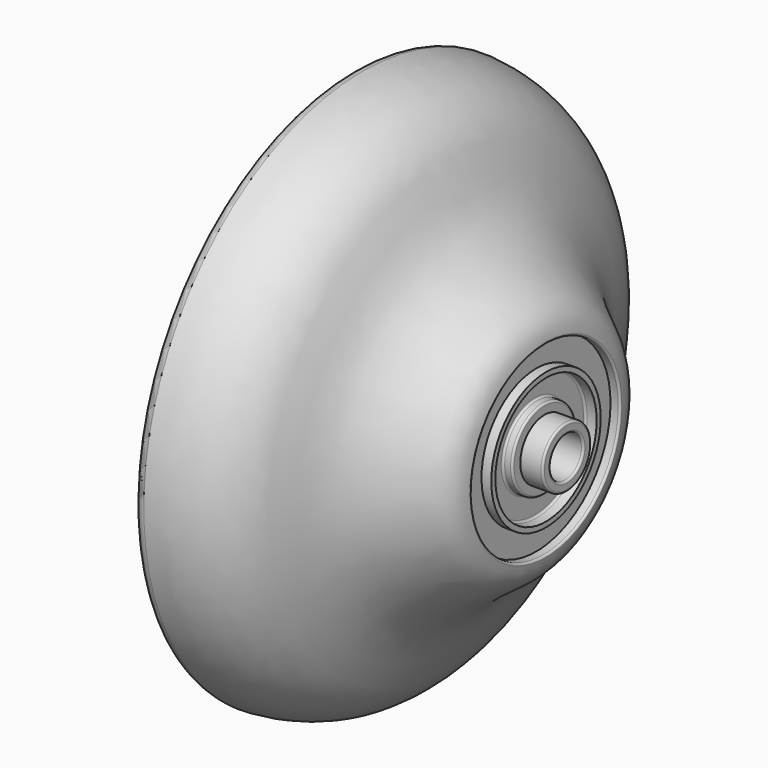
from build123d import *


with BuildPart() as f1:
    # F0 (on Front) → F1 (revolve)
    with BuildSketch(Plane.XZ):
        with BuildLine():
            ThreePointArc((103.2552067209, -7.3173598393), (103.3966280772, -7.2587811955), (103.4552067209, -7.1173598393))
            Line((103.4552067209, -7.1173598393), (103.4552067209, -6.5173598393))
            ThreePointArc((103.4552067209, -6.5173598393), (103.3966280772, -6.3759384831), (103.2552067209, -6.3173598393))
            Line((103.2552067209, -6.3173598393), (101.1552067209, -6.3173598393))
            Line((101.1552067209, -6.3173598393), (101.1552067209, -5.5173598393))
            ThreePointArc((101.1552067209, -5.5173598393), (101.0966280772, -5.3759384831), (100.9552067209, -5.3173598393))
            Line((100.9552067209, -5.3173598393), (100.3552067209, -5.3173598393))
            ThreePointArc((100.3552067209, -5.3173598393), (100.2137853647, -5.2587811955), (100.1552067209, -5.1173598393))
            Line((100.1552067209, -5.1173598393), (100.1552067209, -3.1639273529))
            ThreePointArc((100.1552067209, -3.1639273529), (100.2118270722, -3.0244917895), (100.3496294843, -2.9640051319))
            Line((100.3496294843, -2.9640051319), (101.3047594914, -2.9373598393))
            Line((101.3047594914, -2.9373598393), (101.3047594914, -2.4173411505))
            Line((101.3047594914, -2.4173411505), (100.3047594914, -2.4173411505))
            Line((100.3047594914, -2.4173411505), (100.3047594914, 0.0826588495))
            Line((100.3047594914, 0.0826588495), (101.0992726788, 0.0831378613))
            ThreePointArc((101.0992726788, 0.0831378613), (101.2445709399, 0.1458302845), (101.2988300096, 0.2944838347))
            add(Edge.make_bspline(
                [(101.2988300096, 0.2944838347), (101.1837805651, 2.3192337828), (97.4272016608, 4.3663124435), (92.5835769481, 8.9137634036), (91.1474619441, 15.4833901881), (86.3560860602, 18.3157026115), (82.5253100104, 18.5507547204)],
                knots=[0.0074185875, 0.0074185875, 0.0074185875, 0.0074185875, 0.2246292525, 0.46868406, 0.7055599611, 0.9757749259, 0.9757749259, 0.9757749259, 0.9757749259], degree=3))
            ThreePointArc((82.5253100104, 18.5507547204), (81.7789545345, 18.2810698276), (81.4640663156, 17.5526318774))
            Line((81.4640663156, 17.5526318774), (81.4640663156, 14.1809673676))
            ThreePointArc((81.4640663156, 14.1809673676), (81.6396089198, 13.8005368242), (82.0429759088, 13.6872333541))
            add(Edge.make_bspline(
                [(82.0429759088, 13.6872333541), (83.3930109688, 14.001159411), (86.6538464033, 14.8354332287), (90.3373383246, 9.5329025549), (91.7284265161, 6.6010556184)],
                knots=[0, 0, 0, 0, 0.399832213, 1, 1, 1, 1], degree=3))
            add(Edge.make_bspline(
                [(91.7284265161, 6.6010556184), (95.0950754885, 3.4767219881), (96.7161215521, 0.3852537708), (97.8513108201, -3.8897465019), (98.094652149, -4.9974876869)],
                knots=[0, 0, 0, 0, 0.5613977894, 0.8048382446, 0.8048382446, 0.8048382446, 0.8048382446], degree=3))
            add(Edge.make_bspline(
                [(98.9453257242, -7.1391716953), (98.9111686024, -6.8278420862), (98.8070010851, -6.1078212195), (98.3544529116, -5.3993618529), (98.094652149, -4.9974876869)],
                knots=[0.0760588529, 0.0760588529, 0.0760588529, 0.0760588529, 0.4748405233, 1, 1, 1, 1], degree=3))
            ThreePointArc((98.9453257242, -7.1391716953), (99.0106456417, -7.2662933332), (99.1441327737, -7.3173598393))
            Line((99.1441327737, -7.3173598393), (103.2552067209, -7.3173598393))
        make_face()
    revolve(axis=Axis((92.4640663156, 0, -9.4173411505), (-1, 0, 0)))


solid = f1.part
